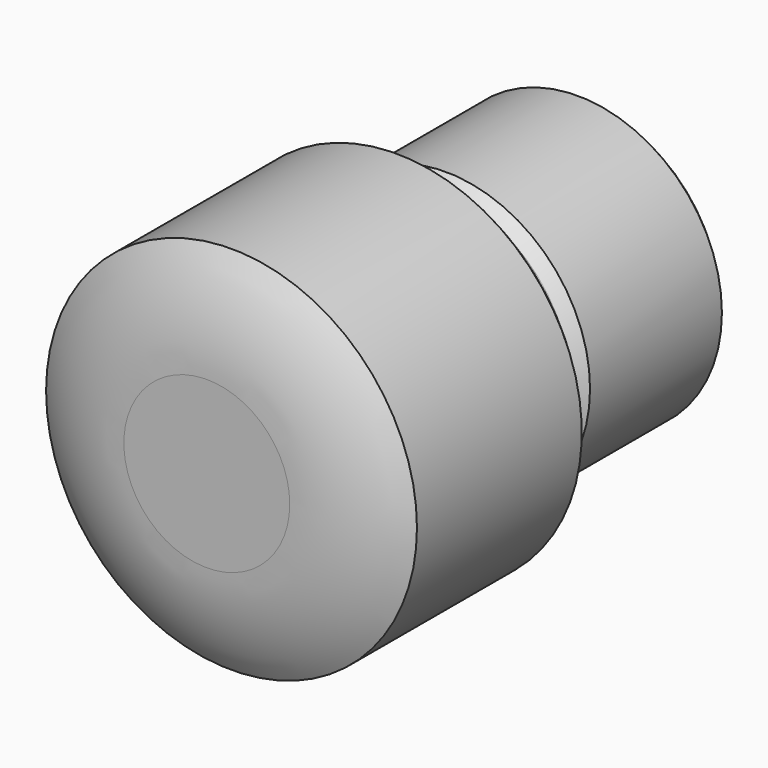
from build123d import *

# Parameters (mm, degrees)
F0_R     = 9
F1_DEPTH = 1.5
F3_R     = 9
F4_DEPTH = 10.5
F5_R     = 6
F6_DEPTH = 2
F7_R     = 7
F8_DEPTH = 9
F9_SIZE  = 0.49999


# Not quite as in the source:
# - a fillet or chamfer that OpenCascade refuses, or shapes differently, is made with other operations: its cross-section is extruded or revolved along the edge and cut away or added
# - a fillet or chamfer is up to 0.001 mm smaller than in the source, because OpenCascade refuses the exact size


with BuildPart() as f1:
    # F0 (on Front) → F1 (new body)
    with BuildSketch(Plane.XZ):
        Circle(F0_R)
    extrude(amount=F1_DEPTH)

    # F2: fillet of radius 9 on 1 edges, made by hand

    # F2_s1 → F2_t2 (revolve, cut)
    with BuildSketch(Plane.XY):
        with BuildLine():
            ThreePointArc((9, 0), (6.6231390258, -1.1168439698), (4.0250628145, -1.5))
            Line((4.0250628145, -1.5), (4.0250628145, -1.68))
            Line((4.0250628145, -1.68), (9, -1.68))
            Line((9, -1.68), (9.18, -1.5))
            ThreePointArc((9.18, -1.5), (9.18, -0.75), (9.0994987437, -0.15))
            Line((9.0994987437, -0.15), (9, 0))
        make_face()
    revolve(axis=Axis((0, -1.5, 0), (0, -1, 0)), mode=Mode.SUBTRACT)

    # F3 (on face) → F4 (join)
    with BuildSketch(Plane(origin=(0, 0, 0), x_dir=(-1, 0, 0), z_dir=(0, 1, 0))):
        Circle(F3_R)
    extrude(amount=F4_DEPTH)

    # F5 (on face) → F6 (join)
    with BuildSketch(Plane(origin=(0, 10.5, 0), x_dir=(-1, 0, 0), z_dir=(0, 1, 0))):
        Circle(F5_R)
    extrude(amount=F6_DEPTH)

    # F7 (on face) → F8 (join)
    with BuildSketch(Plane(origin=(0, 12.5, 0), x_dir=(-1, 0, 0), z_dir=(0, 1, 0))):
        Circle(F7_R)
    extrude(amount=F8_DEPTH)

    # F9 (size 0.5 in the source; OpenCascade refuses exactly that, so slightly less here)
    f9_edges = [f1.edges().sort_by_distance(p)[0] for p in [
        (6, 12.5, 0),
        (6, 10.5, 0),
        (9, 10.5, 0),
        (7, 12.5, 0),
        (7, 21.5, 0),
    ]]
    chamfer(f9_edges, length=F9_SIZE)


solid = f1.part
